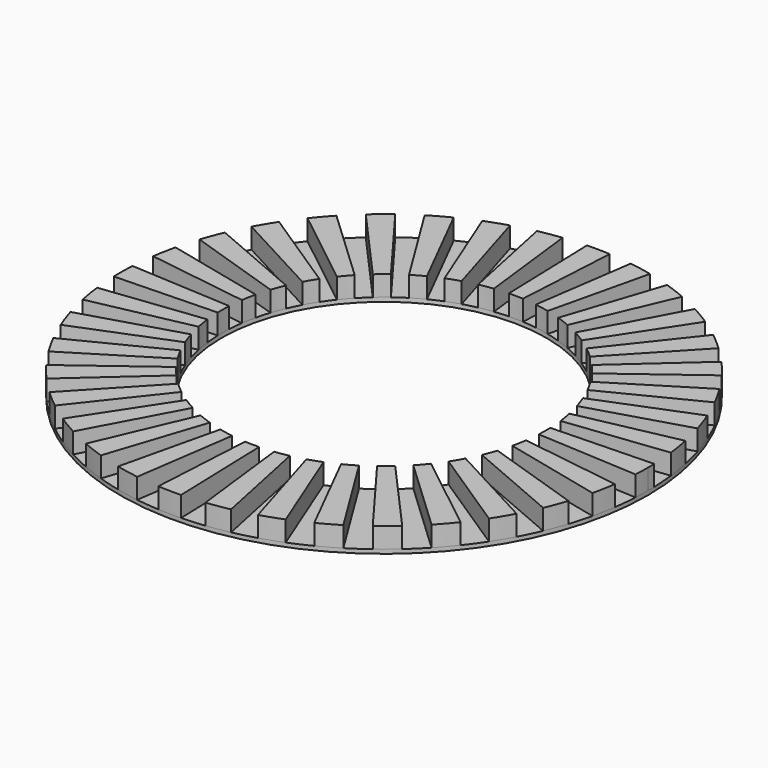
from build123d import *

# Parameters (mm, degrees)
F0_R     = 65
F0_R_2   = 40
F1_DEPTH = 1
F3_DEPTH = 5


# Not quite as in the source:
# - after a boolean that leaves OpenCascade's solid faulty, fix() repairs it


with BuildPart() as f1:
    # F0 (on Top) → F1 (new body)
    with BuildSketch(Plane.XY):
        Circle(F0_R)
        Circle(F0_R_2, mode=Mode.SUBTRACT)
    extrude(amount=F1_DEPTH)

    # F2 (on face) → F3 (join)
    with BuildSketch(Plane.XY.offset(1)):
        with BuildLine():
            Line((-30.7637066326, -57.2590111181), (-18.9315117739, -35.2363145342))
            ThreePointArc((-18.9315117739, -35.2363145342), (-20.4504796225, -34.376996425), (-21.9305188209, -33.4522397493))
            Line((-21.9305188209, -33.4522397493), (-35.637093084, -54.3598895926))
            ThreePointArc((-35.637093084, -54.3598895926), (-33.2320293866, -55.8626191907), (-30.7637066326, -57.2590111181))
        make_face()
        with BuildLine():
            Line((-20.3534138675, -61.731179674), (-12.5251777646, -37.9884182609))
            ThreePointArc((-12.5251777646, -37.9884182609), (-14.1702881022, -37.4059211235), (-15.7884244911, -36.7522196893))
            Line((-15.7884244911, -36.7522196893), (-25.656189798, -59.7223569951))
            ThreePointArc((-25.656189798, -59.7223569951), (-23.0267181661, -60.7846218257), (-20.3534138675, -61.731179674))
        make_face()
        with BuildLine():
            Line((-9.3246929213, -64.3276775729), (-5.738272567, -39.5862631218))
            ThreePointArc((-5.738272567, -39.5862631218), (-7.4595395484, -39.298285837), (-9.1666068724, -38.9355020315))
            Line((-9.1666068724, -38.9355020315), (-14.8957361677, -63.2701908012))
            ThreePointArc((-14.8957361677, -63.2701908012), (-12.1217517662, -63.8597144851), (-9.3246929213, -64.3276775729))
        make_face()
        with BuildLine():
            Line((1.9873541007, -64.9696115402), (1.2229871389, -39.9812994093))
            ThreePointArc((1.2229871389, -39.9812994093), (-0.5221366602, -39.9965920212), (-2.2662665424, -39.9357488468))
            Line((-2.2662665424, -39.9357488468), (-3.6826831315, -64.8955918761))
            ThreePointArc((-3.6826831315, -64.8955918761), (-0.8484720728, -64.9944620344), (1.9873541007, -64.9696115402))
        make_face()
        with BuildLine():
            Line((13.239016374, -63.637476737), (8.1470869994, -39.1615241458))
            ThreePointArc((8.1470869994, -39.1615241458), (6.4311310863, -39.479621996), (4.7029331496, -39.7225681419))
            Line((4.7029331496, -39.7225681419), (7.6422663682, -64.5491732306))
            ThreePointArc((7.6422663682, -64.5491732306), (10.4505880152, -64.1543857436), (13.239016374, -63.637476737))
        make_face()
        with BuildLine():
            Line((24.0884178341, -60.3717494053), (14.8236417441, -37.1518457878))
            ThreePointArc((14.8236417441, -37.1518457878), (13.188992169, -37.7630836342), (11.5292365978, -38.3024373046))
            Line((11.5292365978, -38.3024373046), (18.7350094713, -62.24146062))
            ThreePointArc((18.7350094713, -62.24146062), (21.4321122746, -61.3650109056), (24.0884178341, -60.3717494053))
        make_face()
        with BuildLine():
            Line((34.2059049076, -55.2716570174), (21.0497876354, -34.0133273953))
            ThreePointArc((21.0497876354, -34.0133273953), (19.5461123986, -34.8991330852), (18.0052300259, -35.7185062917))
            Line((18.0052300259, -35.7185062917), (29.2584987921, -58.0425727241))
            ThreePointArc((29.2584987921, -58.0425727241), (31.7624326478, -56.7110912635), (34.2059049076, -55.2716570174))
        make_face()
        with BuildLine():
            Line((43.2840628695, -48.4921632999), (26.6363463812, -29.8413312615))
            ThreePointArc((26.6363463812, -29.8413312615), (25.3093338938, -30.9747900372), (23.9341436508, -32.0492865397))
            Line((23.9341436508, -32.0492865397), (38.8929834326, -52.0800906269))
            ThreePointArc((38.8929834326, -52.0800906269), (41.1276675775, -50.3340338105), (43.2840628695, -48.4921632999))
        make_face()
        with BuildLine():
            Line((51.0470564839, -40.2392597388), (31.4135732209, -24.7626213777))
            ThreePointArc((31.4135732209, -24.7626213777), (30.3035440858, -26.109293668), (29.1358304322, -27.4062654338))
            Line((29.1358304322, -27.4062654338), (47.3457244523, -44.5351813299))
            ThreePointArc((47.3457244523, -44.5351813299), (49.2432591394, -42.4276022105), (51.0470564839, -40.2392597388))
        make_face()
        with BuildLine():
            Line((57.2590111181, -30.7637066326), (35.2363145342, -18.9315117739))
            ThreePointArc((35.2363145342, -18.9315117739), (34.376996425, -20.4504796225), (33.4522397493, -21.9305188209))
            Line((33.4522397493, -21.9305188209), (54.3598895926, -35.637093084))
            ThreePointArc((54.3598895926, -35.637093084), (55.8626191907, -33.2320293866), (57.2590111181, -30.7637066326))
        make_face()
        with BuildLine():
            ThreePointArc((37.9884182609, -12.5251777646), (37.4059211235, -14.1702881022), (36.7522196893, -15.7884244911))
            Line((36.7522196893, -15.7884244911), (59.7223569951, -25.656189798))
            ThreePointArc((59.7223569951, -25.656189798), (60.7846218257, -23.0267181661), (61.731179674, -20.3534138675))
            Line((61.731179674, -20.3534138675), (37.9884182609, -12.5251777646))
        make_face()
        with BuildLine():
            ThreePointArc((39.5862631218, -5.738272567), (39.298285837, -7.4595395484), (38.9355020315, -9.1666068724))
            Line((38.9355020315, -9.1666068724), (63.2701908012, -14.8957361677))
            ThreePointArc((63.2701908012, -14.8957361677), (63.8597144851, -12.1217517662), (64.3276775729, -9.3246929213))
            Line((64.3276775729, -9.3246929213), (39.5862631218, -5.738272567))
        make_face()
        with BuildLine():
            ThreePointArc((40, 0), (39.9839339853, -1.1335885775), (39.9357488468, -2.2662665424))
            Line((39.9357488468, -2.2662665424), (64.8955918761, -3.6826831315))
            ThreePointArc((64.8955918761, -3.6826831315), (64.973892726, -1.8420814384), (65, 0))
            ThreePointArc((65, 0), (64.992402441, 0.9937932104), (64.9696115402, 1.9873541007))
            Line((64.9696115402, 1.9873541007), (39.9812994093, 1.2229871389))
            ThreePointArc((39.9812994093, 1.2229871389), (39.9953245791, 0.6115650525), (40, 0))
        make_face()
        with BuildLine():
            ThreePointArc((39.1615241458, 8.1470869994), (39.479621996, 6.4311310863), (39.7225681419, 4.7029331496))
            Line((39.7225681419, 4.7029331496), (64.5491732306, 7.6422663682))
            ThreePointArc((64.5491732306, 7.6422663682), (64.1543857436, 10.4505880152), (63.637476737, 13.239016374))
            Line((63.637476737, 13.239016374), (39.1615241458, 8.1470869994))
        make_face()
        with BuildLine():
            ThreePointArc((37.1518457878, 14.8236417441), (37.7630836342, 13.188992169), (38.3024373046, 11.5292365978))
            Line((38.3024373046, 11.5292365978), (62.24146062, 18.7350094713))
            ThreePointArc((62.24146062, 18.7350094713), (61.3650109056, 21.4321122746), (60.3717494053, 24.0884178341))
            Line((60.3717494053, 24.0884178341), (37.1518457878, 14.8236417441))
        make_face()
        with BuildLine():
            ThreePointArc((34.0133273953, 21.0497876354), (34.8991330852, 19.5461123986), (35.7185062917, 18.0052300259))
            Line((35.7185062917, 18.0052300259), (58.0425727241, 29.2584987921))
            ThreePointArc((58.0425727241, 29.2584987921), (56.7110912635, 31.7624326478), (55.2716570174, 34.2059049076))
            Line((55.2716570174, 34.2059049076), (34.0133273953, 21.0497876354))
        make_face()
        with BuildLine():
            ThreePointArc((29.8413312615, 26.6363463812), (30.9747900372, 25.3093338938), (32.0492865397, 23.9341436508))
            Line((32.0492865397, 23.9341436508), (52.0800906269, 38.8929834326))
            ThreePointArc((52.0800906269, 38.8929834326), (50.3340338105, 41.1276675775), (48.4921632999, 43.2840628695))
            Line((48.4921632999, 43.2840628695), (29.8413312615, 26.6363463812))
        make_face()
        with BuildLine():
            ThreePointArc((24.7626213777, 31.4135732209), (26.109293668, 30.3035440858), (27.4062654338, 29.1358304322))
            Line((27.4062654338, 29.1358304322), (44.5351813299, 47.3457244523))
            ThreePointArc((44.5351813299, 47.3457244523), (42.4276022105, 49.2432591394), (40.2392597388, 51.0470564839))
            Line((40.2392597388, 51.0470564839), (24.7626213777, 31.4135732209))
        make_face()
        with BuildLine():
            ThreePointArc((18.9315117739, 35.2363145342), (20.4504796225, 34.376996425), (21.9305188209, 33.4522397493))
            Line((21.9305188209, 33.4522397493), (35.637093084, 54.3598895926))
            ThreePointArc((35.637093084, 54.3598895926), (33.2320293866, 55.8626191907), (30.7637066326, 57.2590111181))
            Line((30.7637066326, 57.2590111181), (18.9315117739, 35.2363145342))
        make_face()
        with BuildLine():
            ThreePointArc((12.5251777646, 37.9884182609), (14.1702881022, 37.4059211235), (15.7884244911, 36.7522196893))
            Line((15.7884244911, 36.7522196893), (25.656189798, 59.7223569951))
            ThreePointArc((25.656189798, 59.7223569951), (23.0267181661, 60.7846218257), (20.3534138675, 61.731179674))
            Line((20.3534138675, 61.731179674), (12.5251777646, 37.9884182609))
        make_face()
        with BuildLine():
            ThreePointArc((5.738272567, 39.5862631218), (7.4595395484, 39.298285837), (9.1666068724, 38.9355020315))
            Line((9.1666068724, 38.9355020315), (14.8957361677, 63.2701908012))
            ThreePointArc((14.8957361677, 63.2701908012), (12.1217517662, 63.8597144851), (9.3246929213, 64.3276775729))
            Line((9.3246929213, 64.3276775729), (5.738272567, 39.5862631218))
        make_face()
        with BuildLine():
            ThreePointArc((-1.2229871389, 39.9812994093), (0.5221366602, 39.9965920212), (2.2662665424, 39.9357488468))
            Line((2.2662665424, 39.9357488468), (3.6826831315, 64.8955918761))
            ThreePointArc((3.6826831315, 64.8955918761), (0.8484720728, 64.9944620344), (-1.9873541007, 64.9696115402))
            Line((-1.9873541007, 64.9696115402), (-1.2229871389, 39.9812994093))
        make_face()
        with BuildLine():
            ThreePointArc((-8.1470869994, 39.1615241458), (-6.4311310863, 39.479621996), (-4.7029331496, 39.7225681419))
            Line((-4.7029331496, 39.7225681419), (-7.6422663682, 64.5491732306))
            ThreePointArc((-7.6422663682, 64.5491732306), (-10.4505880152, 64.1543857436), (-13.239016374, 63.637476737))
            Line((-13.239016374, 63.637476737), (-8.1470869994, 39.1615241458))
        make_face()
        with BuildLine():
            ThreePointArc((-14.8236417441, 37.1518457878), (-13.188992169, 37.7630836342), (-11.5292365978, 38.3024373046))
            Line((-11.5292365978, 38.3024373046), (-18.7350094713, 62.24146062))
            ThreePointArc((-18.7350094713, 62.24146062), (-21.4321122746, 61.3650109056), (-24.0884178341, 60.3717494053))
            Line((-24.0884178341, 60.3717494053), (-14.8236417441, 37.1518457878))
        make_face()
        with BuildLine():
            ThreePointArc((-21.0497876354, 34.0133273953), (-19.5461123986, 34.8991330852), (-18.0052300259, 35.7185062917))
            Line((-18.0052300259, 35.7185062917), (-29.2584987921, 58.0425727241))
            ThreePointArc((-29.2584987921, 58.0425727241), (-31.7624326478, 56.7110912635), (-34.2059049076, 55.2716570174))
            Line((-34.2059049076, 55.2716570174), (-21.0497876354, 34.0133273953))
        make_face()
        with BuildLine():
            ThreePointArc((-26.6363463812, 29.8413312615), (-25.3093338938, 30.9747900372), (-23.9341436508, 32.0492865397))
            Line((-23.9341436508, 32.0492865397), (-38.8929834326, 52.0800906269))
            ThreePointArc((-38.8929834326, 52.0800906269), (-41.1276675775, 50.3340338105), (-43.2840628695, 48.4921632999))
            Line((-43.2840628695, 48.4921632999), (-26.6363463812, 29.8413312615))
        make_face()
        with BuildLine():
            ThreePointArc((-31.4135732209, 24.7626213777), (-30.3035440858, 26.109293668), (-29.1358304322, 27.4062654338))
            Line((-29.1358304322, 27.4062654338), (-47.3457244523, 44.5351813299))
            ThreePointArc((-47.3457244523, 44.5351813299), (-49.2432591394, 42.4276022105), (-51.0470564839, 40.2392597388))
            Line((-51.0470564839, 40.2392597388), (-31.4135732209, 24.7626213777))
        make_face()
        with BuildLine():
            ThreePointArc((-35.2363145342, 18.9315117739), (-34.376996425, 20.4504796225), (-33.4522397493, 21.9305188209))
            Line((-33.4522397493, 21.9305188209), (-54.3598895926, 35.637093084))
            ThreePointArc((-54.3598895926, 35.637093084), (-55.8626191907, 33.2320293866), (-57.2590111181, 30.7637066326))
            Line((-57.2590111181, 30.7637066326), (-35.2363145342, 18.9315117739))
        make_face()
        with BuildLine():
            Line((-61.731179674, 20.3534138675), (-37.9884182609, 12.5251777646))
            ThreePointArc((-37.9884182609, 12.5251777646), (-37.4059211235, 14.1702881022), (-36.7522196893, 15.7884244911))
            Line((-36.7522196893, 15.7884244911), (-59.7223569951, 25.656189798))
            ThreePointArc((-59.7223569951, 25.656189798), (-60.7846218257, 23.0267181661), (-61.731179674, 20.3534138675))
        make_face()
        with BuildLine():
            Line((-64.3276775729, 9.3246929213), (-39.5862631218, 5.738272567))
            ThreePointArc((-39.5862631218, 5.738272567), (-39.298285837, 7.4595395484), (-38.9355020315, 9.1666068724))
            Line((-38.9355020315, 9.1666068724), (-63.2701908012, 14.8957361677))
            ThreePointArc((-63.2701908012, 14.8957361677), (-63.8597144851, 12.1217517662), (-64.3276775729, 9.3246929213))
        make_face()
        with BuildLine():
            Line((-64.9696115402, -1.9873541007), (-39.9812994093, -1.2229871389))
            ThreePointArc((-39.9812994093, -1.2229871389), (-39.9965920212, 0.5221366602), (-39.9357488468, 2.2662665424))
            Line((-39.9357488468, 2.2662665424), (-64.8955918761, 3.6826831315))
            ThreePointArc((-64.8955918761, 3.6826831315), (-64.9944620344, 0.8484720728), (-64.9696115402, -1.9873541007))
        make_face()
        with BuildLine():
            Line((-63.637476737, -13.239016374), (-39.1615241458, -8.1470869994))
            ThreePointArc((-39.1615241458, -8.1470869994), (-39.479621996, -6.4311310863), (-39.7225681419, -4.7029331496))
            Line((-39.7225681419, -4.7029331496), (-64.5491732306, -7.6422663682))
            ThreePointArc((-64.5491732306, -7.6422663682), (-64.1543857436, -10.4505880152), (-63.637476737, -13.239016374))
        make_face()
        with BuildLine():
            Line((-60.3717494053, -24.0884178341), (-37.1518457878, -14.8236417441))
            ThreePointArc((-37.1518457878, -14.8236417441), (-37.7630836342, -13.188992169), (-38.3024373046, -11.5292365978))
            Line((-38.3024373046, -11.5292365978), (-62.24146062, -18.7350094713))
            ThreePointArc((-62.24146062, -18.7350094713), (-61.3650109056, -21.4321122746), (-60.3717494053, -24.0884178341))
        make_face()
        with BuildLine():
            Line((-55.2716570174, -34.2059049076), (-34.0133273953, -21.0497876354))
            ThreePointArc((-34.0133273953, -21.0497876354), (-34.8991330852, -19.5461123986), (-35.7185062917, -18.0052300259))
            Line((-35.7185062917, -18.0052300259), (-58.0425727241, -29.2584987921))
            ThreePointArc((-58.0425727241, -29.2584987921), (-56.7110912635, -31.7624326478), (-55.2716570174, -34.2059049076))
        make_face()
        with BuildLine():
            Line((-48.4921632999, -43.2840628695), (-29.8413312615, -26.6363463812))
            ThreePointArc((-29.8413312615, -26.6363463812), (-30.9747900372, -25.3093338938), (-32.0492865397, -23.9341436508))
            Line((-32.0492865397, -23.9341436508), (-52.0800906269, -38.8929834326))
            ThreePointArc((-52.0800906269, -38.8929834326), (-50.3340338105, -41.1276675775), (-48.4921632999, -43.2840628695))
        make_face()
        with BuildLine():
            Line((-40.2392597388, -51.0470564839), (-24.7626213777, -31.4135732209))
            ThreePointArc((-24.7626213777, -31.4135732209), (-26.109293668, -30.3035440858), (-27.4062654338, -29.1358304322))
            Line((-27.4062654338, -29.1358304322), (-44.5351813299, -47.3457244523))
            ThreePointArc((-44.5351813299, -47.3457244523), (-42.4276022105, -49.2432591394), (-40.2392597388, -51.0470564839))
        make_face()
    extrude(amount=F3_DEPTH)

    add(f1.part.fix(), mode=Mode.REPLACE)


solid = f1.part
